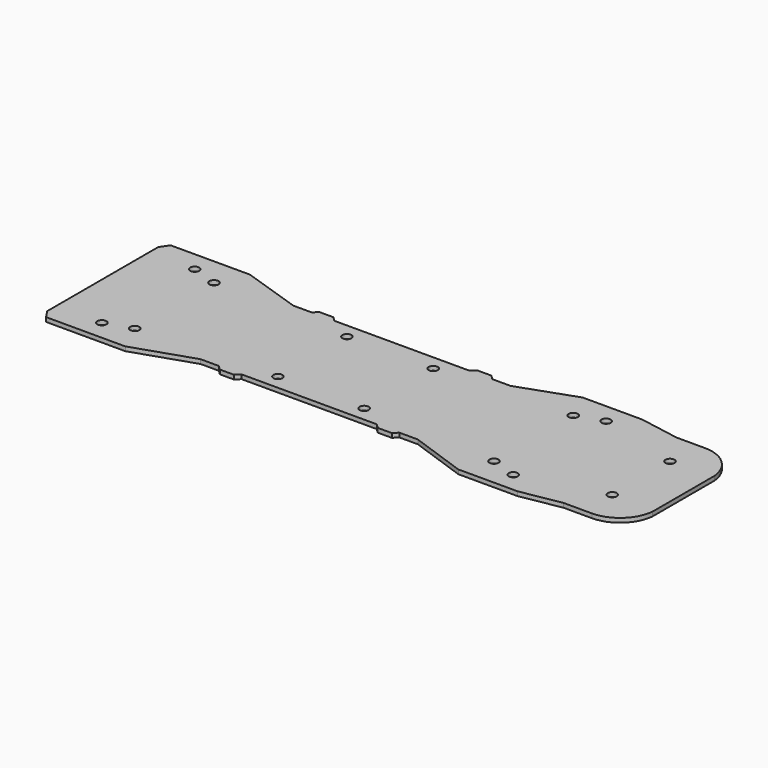
from build123d import *

# Parameters (mm, degrees)
F0_R     = 1.6
F1_DEPTH = 1.5


# Not quite as in the source:
# - ends of sketch curves that miss each other by under 0.0002 mm in the source are joined


with BuildPart() as f1:
    # F0 (on Top) → F1 (new body)
    with BuildSketch(Plane.XY):
        with BuildLine():
            Line((-9.1814305153, -17.5127292487), (-6.6814305153, -17.5127292487))
            Line((-6.6814305153, -17.5127292487), (-5.1814305153, -16.0127292487))
            Line((-5.1814305153, -16.0127292487), (1.3185694847, -16.0127292487))
            Line((1.3185694847, -16.0127292487), (21.2185694847, -23.0127292487))
            Line((21.2185694847, -23.0127292487), (42.2185694847, -23.0127292487))
            Line((42.2185694847, -23.0127292487), (56.4220884847, -20.5127292487))
            Line((56.4220884847, -20.5127292487), (66.4220884847, -20.5127292487))
            ThreePointArc((66.4220884847, -20.5127292487), (74.8259566177, -17.2661070322), (78.864355153, -9.2127293132))
            Line((78.864355153, -9.2127293132), (78.8643544847, 18.1872707513))
            ThreePointArc((78.8643544847, 18.1872707513), (74.8259566177, 26.2406485347), (66.4220884847, 29.4872707513))
            Line((66.4220884847, 29.4872707513), (56.4220884847, 29.4872707513))
            Line((56.4220884847, 29.4872707513), (42.2185694847, 31.9872707513))
            Line((42.2185694847, 31.9872707513), (21.2185694847, 31.9872707513))
            Line((21.2185694847, 31.9872707513), (1.3185694847, 24.9872707513))
            Line((1.3185694847, 24.9872707513), (-5.1814305153, 24.9872707513))
            Line((-5.1814305153, 24.9872707513), (-6.6814305153, 26.4872707513))
            Line((-6.6814305153, 26.4872707513), (-9.1814305153, 26.4872707513))
            Line((-9.1814305153, 26.4872707513), (-11.6814305153, 26.4872707513))
            Line((-11.6814305153, 26.4872707513), (-13.1814305153, 24.9872707513))
            Line((-13.1814305153, 24.9872707513), (-60.9814305153, 24.9872707513))
            Line((-60.9814305153, 24.9872707513), (-62.4814305153, 26.4872707513))
            Line((-62.4814305153, 26.4872707513), (-64.9814305153, 26.4872707513))
            Line((-64.9814305153, 26.4872707513), (-67.4814305153, 26.4872707513))
            Line((-67.4814305153, 26.4872707513), (-68.9814305153, 24.9872707513))
            Line((-68.9814305153, 24.9872707513), (-75.4814305153, 24.9872707513))
            Line((-75.4814305153, 24.9872707513), (-96.4814305153, 31.9872707513))
            Line((-96.4814305153, 31.9872707513), (-116.4814305153, 31.9872707513))
            Line((-116.4814305153, 31.9872707513), (-124.4814305153, 31.9872707513))
            Line((-124.4814305153, 31.9872707513), (-126.4814305153, 28.9872707513))
            Line((-126.4814305153, 28.9872707513), (-126.4814305153, -20.0127292487))
            Line((-126.4814305153, -20.0127292487), (-124.4814305153, -23.0127292487))
            Line((-124.4814305153, -23.0127292487), (-116.4814305153, -23.0127292487))
            Line((-116.4814305153, -23.0127292487), (-96.4814305153, -23.0127292487))
            Line((-96.4814305153, -23.0127292487), (-75.4814305153, -16.0127292487))
            Line((-75.4814305153, -16.0127292487), (-68.9814305153, -16.0127292487))
            Line((-68.9814305153, -16.0127292487), (-67.4814305153, -17.5127292487))
            Line((-67.4814305153, -17.5127292487), (-64.9814305153, -17.5127292487))
            Line((-64.9814305153, -17.5127292487), (-62.4814305153, -17.5127292487))
            Line((-62.4814305153, -17.5127292487), (-60.9814305153, -16.0127292487))
            Line((-60.9814305153, -16.0127292487), (-13.1814305153, -16.0127292487))
            Line((-13.1814305153, -16.0127292487), (-11.6814305153, -17.5127292487))
            Line((-11.6814305153, -17.5127292487), (-9.1814305153, -17.5127292487))
        make_face()
        with Locations((-110.3480007641, -16.0127292487)):
            Circle(F0_R, mode=Mode.SUBTRACT)
        with Locations((-101.1275529865, -13.0127292487)):
            Circle(F0_R, mode=Mode.SUBTRACT)
        with Locations((-52.3314305153, -10.7627292487)):
            Circle(F0_R, mode=Mode.SUBTRACT)
        with Locations((-21.8314305153, -10.7627292487)):
            Circle(F0_R, mode=Mode.SUBTRACT)
        with Locations((25.8646919559, -13.0127292487)):
            Circle(F0_R, mode=Mode.SUBTRACT)
        with Locations((35.0851397335, -16.0127292487)):
            Circle(F0_R, mode=Mode.SUBTRACT)
        with Locations((63.8643544847, -8.2627292487)):
            Circle(F0_R, mode=Mode.SUBTRACT)
        with Locations((-101.1275529865, 21.9872707513)):
            Circle(F0_R, mode=Mode.SUBTRACT)
        with Locations((-110.3480007641, 24.9872707513)):
            Circle(F0_R, mode=Mode.SUBTRACT)
        with Locations((-52.3314305153, 19.7372707513)):
            Circle(F0_R, mode=Mode.SUBTRACT)
        with Locations((63.8643544847, 17.2372707513)):
            Circle(F0_R, mode=Mode.SUBTRACT)
        with Locations((-21.8314305153, 19.7372707513)):
            Circle(F0_R, mode=Mode.SUBTRACT)
        with Locations((25.8646919559, 21.9872707513)):
            Circle(F0_R, mode=Mode.SUBTRACT)
        with Locations((35.0851397335, 24.9872707513)):
            Circle(F0_R, mode=Mode.SUBTRACT)
    extrude(amount=F1_DEPTH)


solid = f1.part
